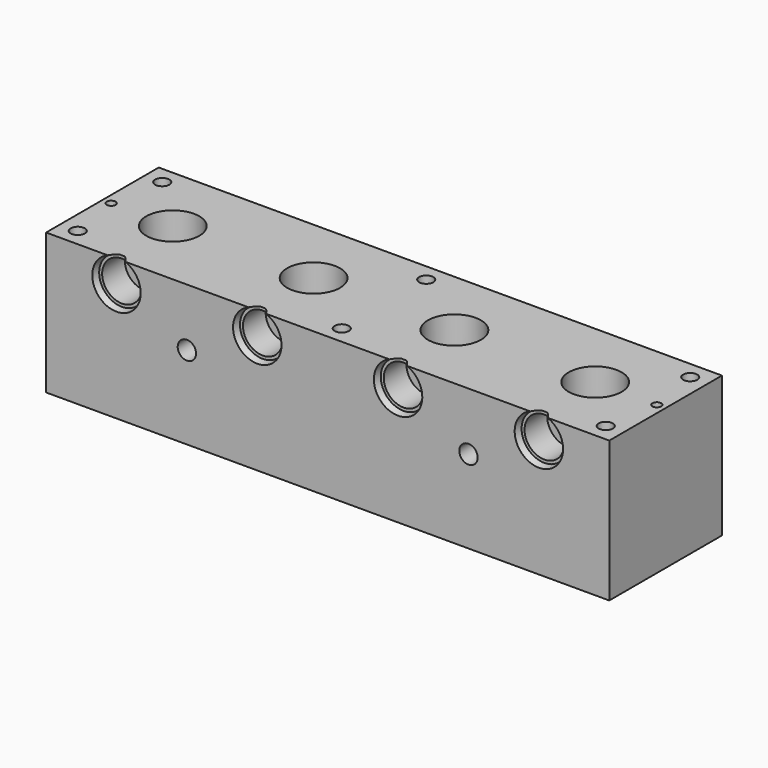
from build123d import *

# Parameters (mm, degrees)
F0_W      = 203.2
F0_H      = 50.8
F1_DEPTH  = 50.8
F2_R      = 6.4135
F3_DEPTH  = 50.801
F5_R      = 9.5631
F6_DEPTH  = 19.05
F7_R      = 4.2452390876
F7_R_2    = 4.1818677439
F7_R_3    = 3.7667127991
F7_R_4    = 4.0342305833
F8_DEPTH  = 16.8318212187
F9_R      = 7.14375
F10_DEPTH = 12.7
F11_R     = 3.3147
F12_DEPTH = 50.801
F13_R     = 2.5527
F14_DEPTH = 25.4
F15_R     = 2.5527
F16_DEPTH = 25.4
F17_R     = 4.7625
F17_R_2   = 4.9964763445
F17_R_3   = 4.6533754175
F17_R_4   = 4.7625013339
F18_DEPTH = 21.3800292737
F19_R     = 8.7757
F19_R_2   = 6.9977
F20_DEPTH = 1.27
F21_R     = 1.5875
F22_DEPTH = 4.7625
F23_R     = 8.7376
F24_DEPTH = 2.4638
F24_TAPER = 12
F25_R     = 7.14375
F26_DEPTH = 13.0048
F27_R     = 8.7376
F28_DEPTH = 2.4638
F28_TAPER = 12


# Not quite as in the source:
# - a feature names something its author has since deleted; it is built from what else it names


with BuildPart() as f1:
    # F0 (on Top) → F1 (new body)
    with BuildSketch(Plane.XY):
        Rectangle(F0_W, F0_H)
    extrude(amount=F1_DEPTH)

    # F2 (on face) → F3 (cut, through all)
    with BuildSketch(Plane.XY.offset(50.8)):
        with Locations((76.2, 0)):
            Circle(F2_R)
        with Locations((25.4, 0)):
            Circle(F2_R)
        with Locations((-25.4, 0)):
            Circle(F2_R)
        with Locations((-76.2, 0)):
            Circle(F2_R)
    extrude(amount=-F3_DEPTH, mode=Mode.SUBTRACT)

    # F5 (on face) → F6 (cut)
    with BuildSketch(Plane.XY.offset(50.8)):
        with Locations((76.2, 0)):
            Circle(F5_R)
        with Locations((25.4, 0)):
            Circle(F5_R)
        with Locations((-25.4, 0)):
            Circle(F5_R)
        with Locations((-76.2, 0)):
            Circle(F5_R)
    extrude(amount=-F6_DEPTH, mode=Mode.SUBTRACT)

    # F7 (on face) → F8 (cut, through all)
    with BuildSketch(Plane.XZ.offset(25.4)):
        with Locations((76.2, 42.6466)):
            Circle(F7_R)
        with Locations((25.4, 42.6466)):
            Circle(F7_R_2)
        with Locations((-25.4, 42.6466)):
            Circle(F7_R_3)
        with Locations((-76.2, 42.6466)):
            Circle(F7_R_4)
    extrude(amount=-F8_DEPTH, mode=Mode.SUBTRACT)

    # F9 (on face) → F10 (cut)
    with BuildSketch(Plane.XZ.offset(25.4)):
        with Locations((76.2, 42.6466)):
            Circle(F9_R)
        with Locations((25.4, 42.6466)):
            Circle(F9_R)
        with Locations((-25.4, 42.6466)):
            Circle(F9_R)
        with Locations((-76.2, 42.6466)):
            Circle(F9_R)
    extrude(amount=-F10_DEPTH, mode=Mode.SUBTRACT)

    # F11 (on face) → F12 (cut, through all)
    with BuildSketch(Plane.XZ.offset(25.4)):
        with Locations((50.8, 29.9466)):
            Circle(F11_R)
        with Locations((-50.8, 29.9466)):
            Circle(F11_R)
    extrude(amount=-F12_DEPTH, mode=Mode.SUBTRACT)

    # F13 (on face) → F14 (cut)
    with BuildSketch(Plane.XY.offset(50.8)):
        with Locations((95.25, 19.05)):
            Circle(F13_R)
        with Locations((95.25, -19.05)):
            Circle(F13_R)
        with Locations((0, -19.05)):
            Circle(F13_R)
        with Locations((0, 19.05)):
            Circle(F13_R)
        with Locations((-95.25, 19.05)):
            Circle(F13_R)
        with Locations((-95.25, -19.05)):
            Circle(F13_R)
    extrude(amount=-F14_DEPTH, mode=Mode.SUBTRACT)

    # F15 (on face) → F16 (cut)
    with BuildSketch(Plane(origin=(0, 0, 0), x_dir=(1, 0, 0), z_dir=(0, 0, -1))):
        with Locations((95.25, 19.05)):
            Circle(F15_R)
        with Locations((95.25, -19.05)):
            Circle(F15_R)
        with Locations((0, -19.05)):
            Circle(F15_R)
        with Locations((0, 19.05)):
            Circle(F15_R)
        with Locations((-95.25, 19.05)):
            Circle(F15_R)
        with Locations((-95.25, -19.05)):
            Circle(F15_R)
    extrude(amount=-F16_DEPTH, mode=Mode.SUBTRACT)

    # F17 (on face) → F18 (cut, through all)
    with BuildSketch(Plane(origin=(0, 25.4, 0), x_dir=(-1, 0, 0), z_dir=(0, 1, 0))):
        with Locations((-76.2, 19.05)):
            Circle(F17_R)
        with Locations((-25.4, 19.05)):
            Circle(F17_R_2)
        with Locations((25.4, 19.05)):
            Circle(F17_R_3)
        with Locations((76.2, 19.05)):
            Circle(F17_R_4)
    extrude(amount=-F18_DEPTH, mode=Mode.SUBTRACT)

    # F19 (on face) → F20 (cut)
    with BuildSketch(Plane.XY.offset(31.75)):
        with Locations((-76.2, 0)):
            Circle(F19_R)
        with Locations((-76.2, 0)):
            Circle(F19_R_2, mode=Mode.SUBTRACT)
        with Locations((-25.1808576286, 0)):
            Circle(F19_R)
        with Locations((-25.1808576286, 0)):
            Circle(F19_R_2, mode=Mode.SUBTRACT)
        with Locations((25.5327448249, 0)):
            Circle(F19_R)
        with Locations((25.5327448249, 0)):
            Circle(F19_R_2, mode=Mode.SUBTRACT)
        with Locations((76.2463510036, 0)):
            Circle(F19_R)
        with Locations((76.2463510036, 0)):
            Circle(F19_R_2, mode=Mode.SUBTRACT)
    extrude(amount=-F20_DEPTH, mode=Mode.SUBTRACT)

    # F21 (on face) → F22 (cut)
    with BuildSketch(Plane.XY.offset(50.8)):
        with Locations((98.425, 0)):
            Circle(F21_R)
        with Locations((-98.425, 0)):
            Circle(F21_R)
    extrude(amount=-F22_DEPTH, mode=Mode.SUBTRACT)

    # F23 (on face) → F24 (cut)
    with BuildSketch(Plane(origin=(0, 25.4, 0), x_dir=(-1, 0, 0), z_dir=(0, 1, 0))):
        with Locations((-76.2, 19.05)):
            Circle(F23_R)
        with Locations((-25.4, 19.05)):
            Circle(F23_R)
        with Locations((25.4, 19.05)):
            Circle(F23_R)
        with Locations((76.2, 19.05)):
            Circle(F23_R)
    extrude(amount=-F24_DEPTH, taper=F24_TAPER, mode=Mode.SUBTRACT)

    # F25 (on face) → F26 (cut)
    with BuildSketch(Plane(origin=(0, 22.9362, 0), x_dir=(-1, 0, 0), z_dir=(0, 1, 0))):
        with Locations((-25.4, 19.05)):
            Circle(F25_R)
        with Locations((-76.2, 19.05)):
            Circle(F25_R)
        with Locations((25.4, 19.05)):
            Circle(F25_R)
        with Locations((76.2, 19.05)):
            Circle(F25_R)
    extrude(amount=-F26_DEPTH, mode=Mode.SUBTRACT)

    # F27 (on face) → F28 (cut)
    with BuildSketch(Plane.XZ.offset(25.4)):
        with Locations((-76.2, 42.6466)):
            Circle(F27_R)
        with Locations((-25.4, 42.6466)):
            Circle(F27_R)
        with Locations((25.4, 42.6466)):
            Circle(F27_R)
        with Locations((76.2, 42.6466)):
            Circle(F27_R)
    extrude(amount=-F28_DEPTH, taper=F28_TAPER, mode=Mode.SUBTRACT)


solid = f1.part
